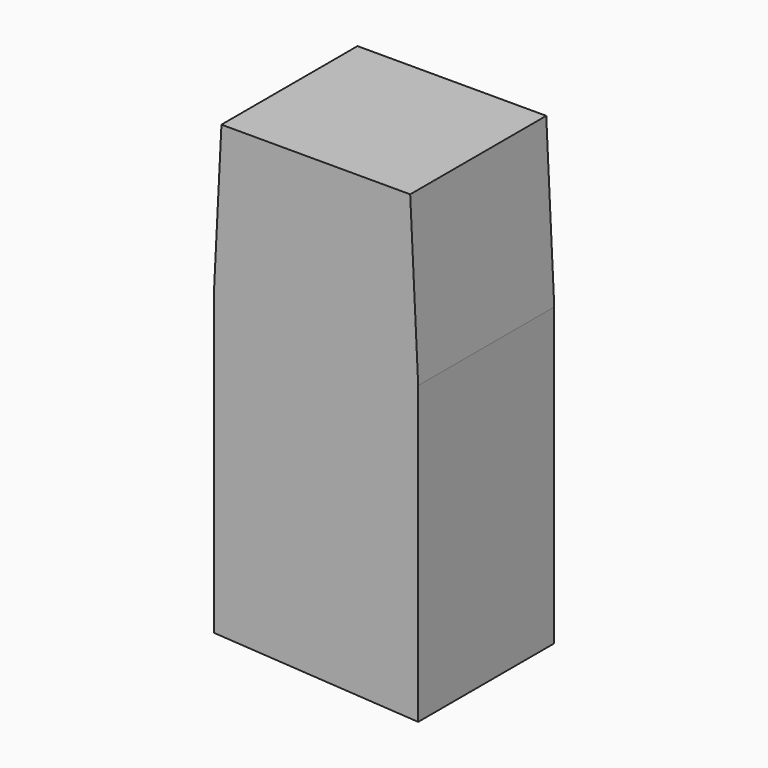
from build123d import *

# Parameters (mm, degrees)
F1_DEPTH = 25.4
F2_DEPTH = 42.9268069565
F3_DEPTH = 118.9797818661


# Not quite as in the source:
# - the program builds the solid bodies; features that only make, move or delete a surface that nothing else refers to are left out


with BuildPart() as f1:
    # F0 (on Front) → F1 (new body)
    with BuildSketch(Plane.XZ):
        Polygon((39.7322513163, -37.4155193567), (36.51605919, 29.1617289186), (-39.3116846681, 29.1617289186), (-42.4041748047, -32.5892791152), align=None)
    extrude(amount=F1_DEPTH)

    # F2 (add): a face of the model
    f2_faces = [f1.faces().sort_by_distance(p)[0] for p in [
        (-0.8911665314, -25.4, -3.3616464638),
    ]]
    extrude(f2_faces, amount=F2_DEPTH)

    # F3 (add): faces of the model
    f3_faces = [f1.faces().sort_by_distance(p)[0] for p in [
        (-1.397812739, -34.1634034783, 29.1617289186),
        (38.1241552532, -34.1634034783, -4.1268952191),
        (-1.3359617442, -34.1634034783, -35.002399236),
    ]]
    extrude(f3_faces, amount=-F3_DEPTH, dir=(0, 0, 1))


solid = f1.part
